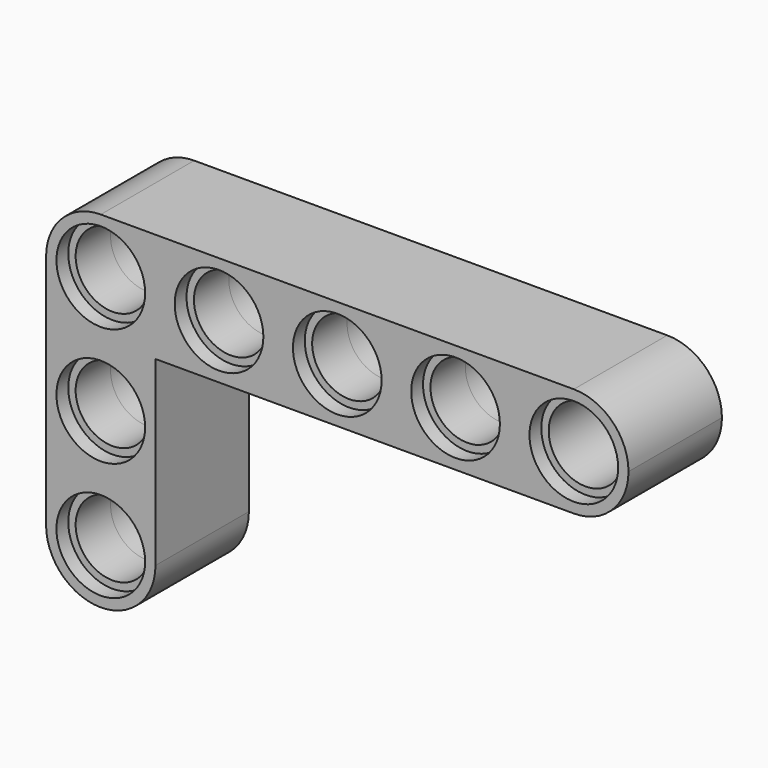
from build123d import *

# Parameters (mm, degrees)
F0_R     = 3
F1_DEPTH = 3.95
F0_R_2   = 2.499
F2_DEPTH = 2.95
F3_R     = 3.69999
F4_R     = 3
F4_W     = 7.4
F4_H     = 7.4
F5_DEPTH = 7.9
F7_R     = 3.69999
F8_R     = 3.7


# Not quite as in the source:
# - a fillet or chamfer is up to 0.001 mm smaller than in the source, because OpenCascade refuses the exact size


with BuildPart() as f1:
    # F0 (on Front) → F1 (new body, symmetric)
    with BuildSketch(Plane.XZ):
        Polygon((19.7, -3.7), (19.7, 3.7), (-19.7, 3.7), (-19.7, -3.7), (-19.7, -19.7), (-12.3, -19.7), (-12.3, -3.7), align=None)
        with Locations((-16, -16)):
            Circle(F0_R, mode=Mode.SUBTRACT)
        with Locations((-16, -8)):
            Circle(F0_R, mode=Mode.SUBTRACT)
        with Locations((-16, 0)):
            Circle(F0_R, mode=Mode.SUBTRACT)
        with Locations((-8, 0)):
            Circle(F0_R, mode=Mode.SUBTRACT)
        Circle(F0_R, mode=Mode.SUBTRACT)
        with Locations((8, 0)):
            Circle(F0_R, mode=Mode.SUBTRACT)
        with Locations((16, 0)):
            Circle(F0_R, mode=Mode.SUBTRACT)
    extrude(amount=F1_DEPTH, both=True)

    # F0 (on Front) → F2 (join, symmetric)
    with BuildSketch(Plane.XZ):
        with Locations((-16, -16)):
            Circle(F0_R)
        with Locations((-16, -16)):
            Circle(F0_R_2, mode=Mode.SUBTRACT)
        with Locations((-16, -8)):
            Circle(F0_R)
        with Locations((-16, -8)):
            Circle(F0_R_2, mode=Mode.SUBTRACT)
        with Locations((-16, 0)):
            Circle(F0_R)
        with Locations((-16, 0)):
            Circle(F0_R_2, mode=Mode.SUBTRACT)
        with Locations((-8, 0)):
            Circle(F0_R)
        with Locations((-8, 0)):
            Circle(F0_R_2, mode=Mode.SUBTRACT)
        Circle(F0_R)
        Circle(F0_R_2, mode=Mode.SUBTRACT)
        with Locations((8, 0)):
            Circle(F0_R)
        with Locations((8, 0)):
            Circle(F0_R_2, mode=Mode.SUBTRACT)
        with Locations((16, 0)):
            Circle(F0_R)
        with Locations((16, 0)):
            Circle(F0_R_2, mode=Mode.SUBTRACT)
    extrude(amount=F2_DEPTH, both=True)

    # F3 (radius 3.7 in the source; OpenCascade refuses exactly that, so slightly less here)
    f3_edges = [f1.edges().sort_by_distance(p)[0] for p in [
        (19.7, 0, 3.7),
        (19.7, 0, -3.7),
    ]]
    fillet(f3_edges, radius=F3_R)

    # F7 (radius 3.7 in the source; OpenCascade refuses exactly that, so slightly less here)
    f7_edges = [f1.edges().sort_by_distance(p)[0] for p in [
        (-12.3, 0, -19.7),
        (-19.7, 0, -19.7),
    ]]
    fillet(f7_edges, radius=F7_R)

    # F8
    f8_edges = [f1.edges().sort_by_distance(p)[0] for p in [
        (-19.7, 0, 3.7),
    ]]
    fillet(f8_edges, radius=F8_R)


with BuildPart() as f5:
    # F4 (on face) → F5 (new body)
    with BuildSketch(Plane.XZ.offset(3.95)):
        Polygon((-12.3, -19.7), (-12.3, -3.7), (-19.7, -3.7), (-19.7, -12.3), (-19.7, -19.7), align=None)
        with Locations((-16, -16)):
            Circle(F4_R, mode=Mode.SUBTRACT)
        with Locations((-16, -8)):
            Circle(F4_R, mode=Mode.SUBTRACT)
        with Locations((-23.4, -16)):
            Rectangle(F4_W, F4_H)
    extrude(amount=F5_DEPTH)


solid = f1.part
